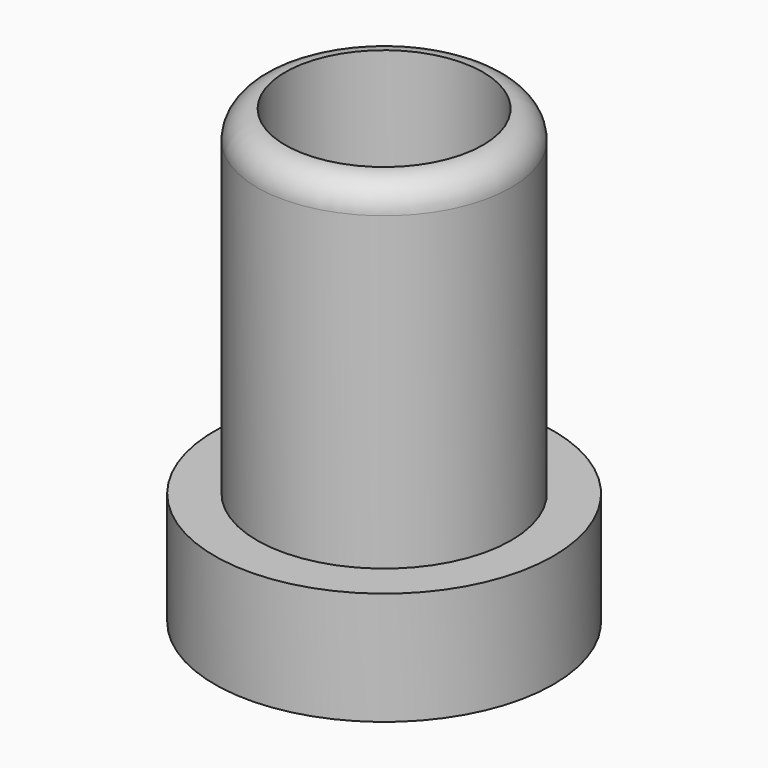
from build123d import *

# Parameters (mm, degrees)
F0_R     = 3
F0_R_2   = 2.25
F1_DEPTH = 2
F0_R_3   = 1.75
F2_DEPTH = 8
F3_R     = 0.5
F4_R     = 0.49999


# Not quite as in the source:
# - a fillet or chamfer is up to 0.001 mm smaller than in the source, because OpenCascade refuses the exact size


with BuildPart() as f1:
    # F0 (on Top) → F1 (new body)
    with BuildSketch(Plane.XY):
        Circle(F0_R)
        Circle(F0_R_2, mode=Mode.SUBTRACT)
    extrude(amount=F1_DEPTH)

    # F0 (on Top) → F2 (join)
    with BuildSketch(Plane.XY):
        Circle(F0_R_2)
        Circle(F0_R_3, mode=Mode.SUBTRACT)
    extrude(amount=F2_DEPTH)

    # F3
    f3_edges = [f1.edges().sort_by_distance(p)[0] for p in [
        (-1.75, 0, 0),
    ]]
    fillet(f3_edges, radius=F3_R)

    # F4 (radius 0.5 in the source; OpenCascade refuses exactly that, so slightly less here)
    f4_edges = [f1.edges().sort_by_distance(p)[0] for p in [
        (-2.25, 0, 8),
    ]]
    fillet(f4_edges, radius=F4_R)


solid = f1.part
